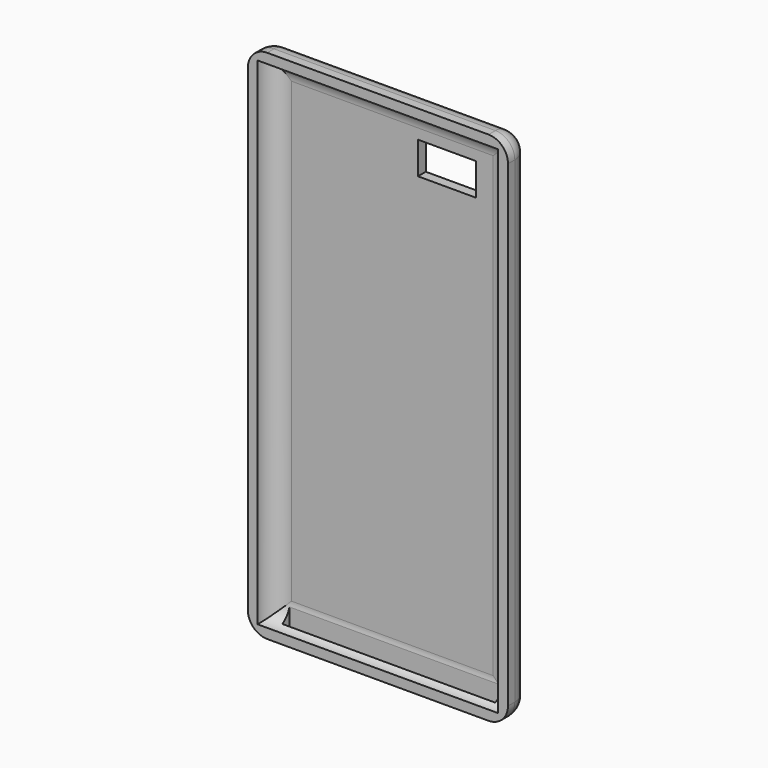
from build123d import *

# Parameters (mm, degrees)
F0_W         = 67.1
F0_H         = 133.1177479803
F1_DEPTH     = 7.2
F2_T         = -2.54
F3_T1_DEPTH  = 123.1177479803
F3_T3_DEPTH  = 57.1
F3_T5_DEPTH  = 14.7
F3_S9_W      = 5.1
F3_S9_H      = 5.1
F3_T10_DEPTH = 5.1
F3_S15_W     = 5.1
F3_S15_H     = 5.1
F3_T16_DEPTH = 5.1
F3_S21_W     = 5.1
F3_S21_H     = 5.1
F3_T22_DEPTH = 5.1
F3_S27_W     = 5.1
F3_S27_H     = 5.1
F3_T28_DEPTH = 5.1
F3_T31_DEPTH = 128.0377479803
F3_T33_DEPTH = 62.02
F3_T39_DEPTH = 140.5088144944
F3_T43_DEPTH = 74.4910665141
F3_T50_DEPTH = 140.5088144944
F3_T54_DEPTH = 74.4910665141
F3_T61_DEPTH = 74.4910665141
F3_T65_DEPTH = 140.5088144944
F3_T72_DEPTH = 74.4910665141
F3_T76_DEPTH = 140.5088144944
F4_W         = 14.9180325679
F4_H         = 8.3196759224
F5_DEPTH     = 12.5
F6_W         = 54.943443346
F6_H         = 2.2745899577
F7_DEPTH     = 12.5


# Not quite as in the source:
# - a fillet or chamfer that OpenCascade refuses, or shapes differently, is made with other operations: its cross-section is extruded or revolved along the edge and cut away or added


with BuildPart() as f1:
    # F0 (on Front) → F1 (new body)
    with BuildSketch(Plane.XZ):
        Rectangle(F0_W, F0_H)
    extrude(amount=F1_DEPTH)

    # F2
    f2_openings = [f1.faces().sort_by_distance(p)[0] for p in [
        (0, -7.2, 0),
    ]]
    offset(amount=F2_T, openings=f2_openings)

    # F3: fillet of radius 5 on 12 edges, made by hand

    # F3_s2 → F3_t1 (cut)
    with BuildSketch(Plane.XY.offset(-61.5588739901)):
        with BuildLine():
            ThreePointArc((-33.55, -5), (-32.0855339059, -1.4644660941), (-28.55, 0))
            Line((-28.55, 0), (-28.55, 0.1))
            Line((-28.55, 0.1), (-33.65, 0.1))
            Line((-33.65, 0.1), (-33.65, -5))
            Line((-33.65, -5), (-33.55, -5))
        make_face()
        with BuildLine():
            ThreePointArc((33.55, -5), (32.0855339059, -1.4644660941), (28.55, 0))
            Line((28.55, 0), (28.55, 0.1))
            Line((28.55, 0.1), (33.65, 0.1))
            Line((33.65, 0.1), (33.65, -5))
            Line((33.65, -5), (33.55, -5))
        make_face()
    extrude(amount=F3_T1_DEPTH, mode=Mode.SUBTRACT)

    # F3_s4 → F3_t3 (cut)
    with BuildSketch(Plane.YZ.offset(-28.55)):
        with BuildLine():
            ThreePointArc((-5, -66.5588739901), (-1.4644660941, -65.0944078961), (0, -61.5588739901))
            Line((0, -61.5588739901), (0.1, -61.5588739901))
            Line((0.1, -61.5588739901), (0.1, -66.6588739901))
            Line((0.1, -66.6588739901), (-5, -66.6588739901))
            Line((-5, -66.6588739901), (-5, -66.5588739901))
        make_face()
        with BuildLine():
            ThreePointArc((-5, 66.5588739901), (-1.4644660941, 65.0944078961), (0, 61.5588739901))
            Line((0, 61.5588739901), (0.1, 61.5588739901))
            Line((0.1, 61.5588739901), (0.1, 66.6588739901))
            Line((0.1, 66.6588739901), (-5, 66.6588739901))
            Line((-5, 66.6588739901), (-5, 66.5588739901))
        make_face()
    extrude(amount=F3_T3_DEPTH, mode=Mode.SUBTRACT)

    # F3_s6 → F3_t5 (cut)
    with BuildSketch(Plane.XZ.offset(5)):
        with BuildLine():
            ThreePointArc((33.55, 61.5588739901), (32.0855339059, 65.0944078961), (28.55, 66.5588739901))
            Line((28.55, 66.5588739901), (28.55, 66.6588739901))
            Line((28.55, 66.6588739901), (33.65, 66.6588739901))
            Line((33.65, 66.6588739901), (33.65, 61.5588739901))
            Line((33.65, 61.5588739901), (33.55, 61.5588739901))
        make_face()
        with BuildLine():
            ThreePointArc((-33.55, 61.5588739901), (-32.0855339059, 65.0944078961), (-28.55, 66.5588739901))
            Line((-28.55, 66.5588739901), (-28.55, 66.6588739901))
            Line((-28.55, 66.6588739901), (-33.65, 66.6588739901))
            Line((-33.65, 66.6588739901), (-33.65, 61.5588739901))
            Line((-33.65, 61.5588739901), (-33.55, 61.5588739901))
        make_face()
        with BuildLine():
            ThreePointArc((-33.55, -61.5588739901), (-32.0855339059, -65.0944078961), (-28.55, -66.5588739901))
            Line((-28.55, -66.5588739901), (-28.55, -66.6588739901))
            Line((-28.55, -66.6588739901), (-33.65, -66.6588739901))
            Line((-33.65, -66.6588739901), (-33.65, -61.5588739901))
            Line((-33.65, -61.5588739901), (-33.55, -61.5588739901))
        make_face()
        with BuildLine():
            ThreePointArc((28.55, -66.5588739901), (32.0855339059, -65.0944078961), (33.55, -61.5588739901))
            Line((33.55, -61.5588739901), (33.65, -61.5588739901))
            Line((33.65, -61.5588739901), (33.65, -66.6588739901))
            Line((33.65, -66.6588739901), (28.55, -66.6588739901))
            Line((28.55, -66.6588739901), (28.55, -66.5588739901))
        make_face()
    extrude(amount=F3_T5_DEPTH, mode=Mode.SUBTRACT)


with BuildPart() as f3_tool8:
    # F3_s9 → F3_t10 (new body)
    with BuildSketch(Plane.YZ.offset(-28.55)):
        with Locations((-2.45, 64.1088739901)):
            Rectangle(F3_S9_W, F3_S9_H)
    extrude(amount=-F3_T10_DEPTH)

    # F3_s11 → F3_t12 (revolve, cut)
    with BuildSketch(Plane(origin=(-28.55, -5, 61.5588739901), x_dir=(0, -0.7071067812, -0.7071067812), z_dir=(0, 0.7071067812, -0.7071067812))):
        with BuildLine():
            ThreePointArc((0, -5), (5, 0), (0, 5))
            Line((0, 5), (0, -5))
        make_face()
    revolve(axis=Axis((-28.55, -5, 61.5588739901), (-1, 0, 0)), mode=Mode.SUBTRACT)


with BuildPart() as f1_1:
    add(f1.part)

    # F3_t7: cut F3_tool8
    add(f3_tool8.part, mode=Mode.SUBTRACT)


with BuildPart() as f3_tool14:
    # F3_s15 → F3_t16 (new body)
    with BuildSketch(Plane.YZ.offset(-28.55)):
        with Locations((-2.45, -64.1088739901)):
            Rectangle(F3_S15_W, F3_S15_H)
    extrude(amount=-F3_T16_DEPTH)

    # F3_s17 → F3_t18 (revolve, cut)
    with BuildSketch(Plane(origin=(-28.55, -5, -61.5588739901), x_dir=(0, -0.7071067812, 0.7071067812), z_dir=(0, -0.7071067812, -0.7071067812))):
        with BuildLine():
            ThreePointArc((0, -5), (5, 0), (0, 5))
            Line((0, 5), (0, -5))
        make_face()
    revolve(axis=Axis((-28.55, -5, -61.5588739901), (-1, 0, 0)), mode=Mode.SUBTRACT)


with BuildPart() as f1_2:
    add(f1_1.part)

    # F3_t13: cut F3_tool14
    add(f3_tool14.part, mode=Mode.SUBTRACT)


with BuildPart() as f3_tool20:
    # F3_s21 → F3_t22 (new body)
    with BuildSketch(Plane.XY.offset(-61.5588739901)):
        with Locations((31.1, -2.45)):
            Rectangle(F3_S21_W, F3_S21_H)
    extrude(amount=-F3_T22_DEPTH)

    # F3_s23 → F3_t24 (revolve, cut)
    with BuildSketch(Plane(origin=(28.55, -5, -61.5588739901), x_dir=(-0.7071067812, -0.7071067812, 0), z_dir=(0.7071067812, -0.7071067812, 0))):
        with BuildLine():
            ThreePointArc((0, -5), (5, 0), (0, 5))
            Line((0, 5), (0, -5))
        make_face()
    revolve(axis=Axis((28.55, -5, -61.5588739901), (0, 0, -1)), mode=Mode.SUBTRACT)


with BuildPart() as f1_3:
    add(f1_2.part)

    # F3_t19: cut F3_tool20
    add(f3_tool20.part, mode=Mode.SUBTRACT)


with BuildPart() as f3_tool26:
    # F3_s27 → F3_t28 (new body)
    with BuildSketch(Plane.YZ.offset(28.55)):
        with Locations((-2.45, 64.1088739901)):
            Rectangle(F3_S27_W, F3_S27_H)
    extrude(amount=F3_T28_DEPTH)

    # F3_s29 → F3_t30 (revolve, cut)
    with BuildSketch(Plane(origin=(28.55, -5, 61.5588739901), x_dir=(0, -0.7071067812, -0.7071067812), z_dir=(0, -0.7071067812, 0.7071067812))):
        with BuildLine():
            ThreePointArc((0, -5), (5, 0), (0, 5))
            Line((0, 5), (0, -5))
        make_face()
    revolve(axis=Axis((28.55, -5, 61.5588739901), (1, 0, 0)), mode=Mode.SUBTRACT)


with BuildPart() as f1_4:
    add(f1_3.part)

    # F3_t25: cut F3_tool26
    add(f3_tool26.part, mode=Mode.SUBTRACT)

    # F3_s32 → F3_t31 (join)
    with BuildSketch(Plane.XY.offset(-64.0188739901)):
        with BuildLine():
            ThreePointArc((-31.01, -7.2), (-29.4347830275, -3.8862348187), (-26.0215733943, -2.54))
            Line((-26.0215733943, -2.54), (-26.0215733943, -2.44))
            Line((-26.0215733943, -2.44), (-31.01, -2.44))
            Line((-31.01, -2.44), (-31.11, -2.54))
            ThreePointArc((-31.11, -2.54), (-31.11, -4.87), (-31.1097685321, -7.1932))
            Line((-31.1097685321, -7.1932), (-31.01, -7.2))
        make_face()
        with BuildLine():
            ThreePointArc((31.01, -7.2), (29.4347830275, -3.8862348187), (26.0215733943, -2.54))
            Line((26.0215733943, -2.54), (26.0215733943, -2.44))
            Line((26.0215733943, -2.44), (31.01, -2.44))
            Line((31.01, -2.44), (31.11, -2.54))
            ThreePointArc((31.11, -2.54), (31.11, -4.87), (31.1097685321, -7.1932))
            Line((31.1097685321, -7.1932), (31.01, -7.2))
        make_face()
    extrude(amount=F3_T31_DEPTH)

    # F3_s34 → F3_t33 (join)
    with BuildSketch(Plane.YZ.offset(-31.01)):
        with BuildLine():
            ThreePointArc((-7.2, -64.0188739901), (-3.8862348187, -62.4436570177), (-2.54, -59.0304473845))
            Line((-2.54, -59.0304473845), (-2.44, -59.0304473845))
            Line((-2.44, -59.0304473845), (-2.44, -64.0188739901))
            Line((-2.44, -64.0188739901), (-2.54, -64.1188739901))
            ThreePointArc((-2.54, -64.1188739901), (-4.87, -64.1188739901), (-7.1932, -64.1186425223))
            Line((-7.1932, -64.1186425223), (-7.2, -64.0188739901))
        make_face()
        with BuildLine():
            ThreePointArc((-7.2, 64.0188739901), (-3.8862348187, 62.4436570177), (-2.54, 59.0304473845))
            Line((-2.54, 59.0304473845), (-2.44, 59.0304473845))
            Line((-2.44, 59.0304473845), (-2.44, 64.0188739901))
            Line((-2.44, 64.0188739901), (-2.54, 64.1188739901))
            ThreePointArc((-2.54, 64.1188739901), (-4.87, 64.1188739901), (-7.1932, 64.1186425223))
            Line((-7.1932, 64.1186425223), (-7.2, 64.0188739901))
        make_face()
    extrude(amount=F3_T33_DEPTH)


with BuildPart() as f3_tool37:
    # F3_s38 → F3_t39 (new body)
    with BuildSketch(Plane.XY.offset(76.4899405043)):
        with BuildLine():
            ThreePointArc((-31.01, -7.2), (-29.4347830275, -3.8862348187), (-26.0215733943, -2.54))
            Line((-26.0215733943, -2.54), (-26.0215733943, -2.44))
            Line((-26.0215733943, -2.44), (-31.01, -2.44))
            Line((-31.01, -2.44), (-31.11, -2.54))
            ThreePointArc((-31.11, -2.54), (-31.11, -4.87), (-31.1097685321, -7.1932))
            Line((-31.1097685321, -7.1932), (-31.01, -7.2))
        make_face()
    extrude(amount=-F3_T39_DEPTH)

    split(bisect_by=Plane.XY.offset(64.0188739901), keep=Keep.TOP)


with BuildPart() as f3_tool41:
    # F3_s42 → F3_t43 (new body)
    with BuildSketch(Plane.YZ.offset(31.01)):
        with BuildLine():
            ThreePointArc((-7.2, 64.0188739901), (-3.8862348187, 62.4436570177), (-2.54, 59.0304473845))
            Line((-2.54, 59.0304473845), (-2.44, 59.0304473845))
            Line((-2.44, 59.0304473845), (-2.44, 64.0188739901))
            Line((-2.44, 64.0188739901), (-2.54, 64.1188739901))
            ThreePointArc((-2.54, 64.1188739901), (-4.87, 64.1188739901), (-7.1932, 64.1186425223))
            Line((-7.1932, 64.1186425223), (-7.2, 64.0188739901))
        make_face()
    extrude(amount=-F3_T43_DEPTH)

    split(bisect_by=Plane.YZ.offset(-31.01), keep=Keep.BOTTOM)


with BuildPart() as f3_tool37_1:
    add(f3_tool37.part)

    # F3_t45: intersect F3_tool41
    add(f3_tool41.part, mode=Mode.INTERSECT)


with BuildPart() as f1_5:
    add(f1_4.part)

    # F3_t35: union F3_tool37
    add(f3_tool37_1.part)


with BuildPart() as f3_tool48:
    # F3_s49 → F3_t50 (new body)
    with BuildSketch(Plane.XY.offset(64.0188739901)):
        with BuildLine():
            ThreePointArc((-31.01, -7.2), (-29.4347830275, -3.8862348187), (-26.0215733943, -2.54))
            Line((-26.0215733943, -2.54), (-26.0215733943, -2.44))
            Line((-26.0215733943, -2.44), (-31.01, -2.44))
            Line((-31.01, -2.44), (-31.11, -2.54))
            ThreePointArc((-31.11, -2.54), (-31.11, -4.87), (-31.1097685321, -7.1932))
            Line((-31.1097685321, -7.1932), (-31.01, -7.2))
        make_face()
    extrude(amount=-F3_T50_DEPTH)

    split(bisect_by=Plane.XY.offset(-64.0188739901), keep=Keep.BOTTOM)


with BuildPart() as f3_tool52:
    # F3_s53 → F3_t54 (new body)
    with BuildSketch(Plane.YZ.offset(-43.4810665141)):
        with BuildLine():
            ThreePointArc((-7.2, -64.0188739901), (-3.8862348187, -62.4436570177), (-2.54, -59.0304473845))
            Line((-2.54, -59.0304473845), (-2.44, -59.0304473845))
            Line((-2.44, -59.0304473845), (-2.44, -64.0188739901))
            Line((-2.44, -64.0188739901), (-2.54, -64.1188739901))
            ThreePointArc((-2.54, -64.1188739901), (-4.87, -64.1188739901), (-7.1932, -64.1186425223))
            Line((-7.1932, -64.1186425223), (-7.2, -64.0188739901))
        make_face()
    extrude(amount=F3_T54_DEPTH)

    split(bisect_by=Plane.YZ.offset(-31.01), keep=Keep.BOTTOM)


with BuildPart() as f3_tool48_1:
    add(f3_tool48.part)

    # F3_t56: intersect F3_tool52
    add(f3_tool52.part, mode=Mode.INTERSECT)


with BuildPart() as f1_6:
    add(f1_5.part)

    # F3_t46: union F3_tool48
    add(f3_tool48_1.part)


with BuildPart() as f3_tool59:
    # F3_s60 → F3_t61 (new body)
    with BuildSketch(Plane.YZ.offset(-31.01)):
        with BuildLine():
            ThreePointArc((-7.2, -64.0188739901), (-3.8862348187, -62.4436570177), (-2.54, -59.0304473845))
            Line((-2.54, -59.0304473845), (-2.44, -59.0304473845))
            Line((-2.44, -59.0304473845), (-2.44, -64.0188739901))
            Line((-2.44, -64.0188739901), (-2.54, -64.1188739901))
            ThreePointArc((-2.54, -64.1188739901), (-4.87, -64.1188739901), (-7.1932, -64.1186425223))
            Line((-7.1932, -64.1186425223), (-7.2, -64.0188739901))
        make_face()
    extrude(amount=F3_T61_DEPTH)

    split(bisect_by=Plane.YZ.offset(31.01), keep=Keep.TOP)


with BuildPart() as f3_tool63:
    # F3_s64 → F3_t65 (new body)
    with BuildSketch(Plane.XY.offset(-76.4899405043)):
        with BuildLine():
            ThreePointArc((31.01, -7.2), (29.4347830275, -3.8862348187), (26.0215733943, -2.54))
            Line((26.0215733943, -2.54), (26.0215733943, -2.44))
            Line((26.0215733943, -2.44), (31.01, -2.44))
            Line((31.01, -2.44), (31.11, -2.54))
            ThreePointArc((31.11, -2.54), (31.11, -4.87), (31.1097685321, -7.1932))
            Line((31.1097685321, -7.1932), (31.01, -7.2))
        make_face()
    extrude(amount=F3_T65_DEPTH)

    split(bisect_by=Plane.XY.offset(-64.0188739901), keep=Keep.BOTTOM)


with BuildPart() as f3_tool59_1:
    add(f3_tool59.part)

    # F3_t67: intersect F3_tool63
    add(f3_tool63.part, mode=Mode.INTERSECT)


with BuildPart() as f1_7:
    add(f1_6.part)

    # F3_t57: union F3_tool59
    add(f3_tool59_1.part)


with BuildPart() as f3_tool70:
    # F3_s71 → F3_t72 (new body)
    with BuildSketch(Plane.YZ.offset(43.4810665141)):
        with BuildLine():
            ThreePointArc((-7.2, 64.0188739901), (-3.8862348187, 62.4436570177), (-2.54, 59.0304473845))
            Line((-2.54, 59.0304473845), (-2.44, 59.0304473845))
            Line((-2.44, 59.0304473845), (-2.44, 64.0188739901))
            Line((-2.44, 64.0188739901), (-2.54, 64.1188739901))
            ThreePointArc((-2.54, 64.1188739901), (-4.87, 64.1188739901), (-7.1932, 64.1186425223))
            Line((-7.1932, 64.1186425223), (-7.2, 64.0188739901))
        make_face()
    extrude(amount=-F3_T72_DEPTH)

    split(bisect_by=Plane.YZ.offset(31.01), keep=Keep.TOP)


with BuildPart() as f3_tool74:
    # F3_s75 → F3_t76 (new body)
    with BuildSketch(Plane.XY.offset(-64.0188739901)):
        with BuildLine():
            ThreePointArc((31.01, -7.2), (29.4347830275, -3.8862348187), (26.0215733943, -2.54))
            Line((26.0215733943, -2.54), (26.0215733943, -2.44))
            Line((26.0215733943, -2.44), (31.01, -2.44))
            Line((31.01, -2.44), (31.11, -2.54))
            ThreePointArc((31.11, -2.54), (31.11, -4.87), (31.1097685321, -7.1932))
            Line((31.1097685321, -7.1932), (31.01, -7.2))
        make_face()
    extrude(amount=F3_T76_DEPTH)

    split(bisect_by=Plane.XY.offset(64.0188739901), keep=Keep.TOP)


with BuildPart() as f3_tool70_1:
    add(f3_tool70.part)

    # F3_t78: intersect F3_tool74
    add(f3_tool74.part, mode=Mode.INTERSECT)


with BuildPart() as f1_8:
    add(f1_7.part)

    # F3_t68: union F3_tool70
    add(f3_tool70_1.part)

    # F4 (on face) → F5 (cut, symmetric)
    with BuildSketch(Plane.XZ.offset(2.54)):
        with Locations((14.0573775861, 52.2131174803)):
            Rectangle(F4_W, F4_H)
    extrude(amount=F5_DEPTH, both=True, mode=Mode.SUBTRACT)

    # F6 (on face) → F7 (cut, symmetric)
    with BuildSketch(Plane(origin=(0, 0, -66.5588739901), x_dir=(1, 0, 0), z_dir=(0, 0, -1))):
        with Locations((1.078278327, 3.8627050212)):
            Rectangle(F6_W, F6_H)
    extrude(amount=F7_DEPTH, both=True, mode=Mode.SUBTRACT)


solid = f1_8.part
